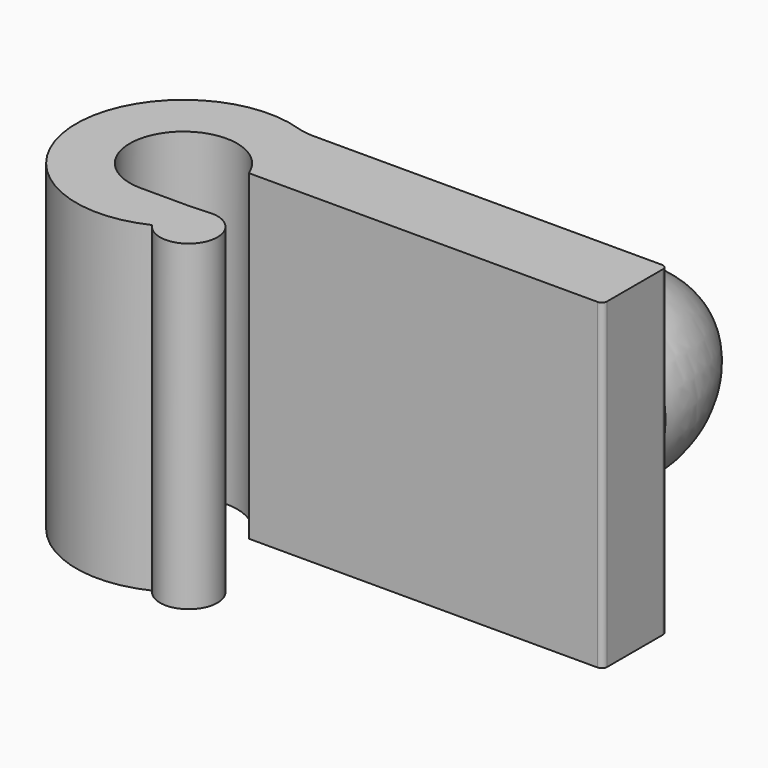
from build123d import *

# Parameters (mm, degrees)
F1_DEPTH      = 6
F3_ANGLE_BACK = 90
F3_ANGLE      = 180


with BuildPart() as f1:
    # F0 (on Top) → F1 (new body, symmetric)
    with BuildSketch(Plane.XY):
        with BuildLine():
            ThreePointArc((0, -2), (-1.6442370944, 1.1386326789), (1.8721820875, 0.7035156225))
            Line((1.8721820875, 0.7035156225), (14.8721820875, 0.7035156225))
            ThreePointArc((14.8721820875, 0.7035156225), (15.0136034438, 0.7620942663), (15.0721820875, 0.9035156225))
            Line((15.0721820875, 0.9035156225), (15.0721820875, 3.5035156225))
            ThreePointArc((15.0721820875, 3.5035156225), (15.0136034438, 3.6449369788), (14.8721820875, 3.7035156225))
            Line((14.8721820875, 3.7035156225), (1.862769321, 3.7035156225))
            ThreePointArc((1.862769321, 3.7035156225), (1.5483999112, 3.7283771782), (1.241846214, 3.8023437484))
            ThreePointArc((1.241846214, 3.8023437484), (-3.9916974669, -0.2575875245), (1.7202481264, -3.6111973615))
            ThreePointArc((1.7202481264, -3.6111973615), (3.5326583833, -3.5785651754), (2.7160516219, -1.9602175008))
            Line((2.7160516219, -1.9602175008), (1.7683124133, -2))
            Line((1.7683124133, -2), (0, -2))
        make_face()
        with BuildLine():
            ThreePointArc((1.7372298538, -3.603058761), (1.7287437795, -3.6071380546), (1.7202481264, -3.6111973615))
            ThreePointArc((1.7202481264, -3.6111973615), (1.7150951564, -3.6032338331), (1.7100129663, -3.5952249487))
            ThreePointArc((1.7100129663, -3.5952249487), (1.7338791511, -3.5635035507), (1.7372298538, -3.603058761))
        make_face(mode=Mode.SUBTRACT)
        with BuildLine():
            ThreePointArc((1.7100129663, -3.5952249487), (1.7150951564, -3.6032338331), (1.7202481264, -3.6111973615))
            ThreePointArc((1.7202481264, -3.6111973615), (1.7287437795, -3.6071380546), (1.7372298538, -3.603058761))
            ThreePointArc((1.7372298538, -3.603058761), (1.7338791511, -3.5635035507), (1.7100129663, -3.5952249487))
        make_face()
    extrude(amount=F1_DEPTH, both=True)



with BuildPart() as f3:
    # F2 (on Top) → F3 (revolve)
    with BuildSketch(Plane.XY, mode=Mode.PRIVATE) as f3_sk:
        with BuildLine():
            Line((7.0616400183, 3.641272106), (9.5616400183, 3.641272106))
            Line((9.5616400183, 3.641272106), (9.5616400183, 10.641272106))
            ThreePointArc((9.5616400183, 10.641272106), (6.8992694056, 8.4986944736), (6.2616400183, 5.141272106))
            Line((6.2616400183, 5.141272106), (7.0616400183, 5.141272106))
            Line((7.0616400183, 5.141272106), (7.0616400183, 3.641272106))
        make_face()
    revolve(f3_sk.sketch.rotate(Axis((9.5616400183, 7.141272106, 0), (0, 1, 0)), -F3_ANGLE_BACK), axis=Axis((9.5616400183, 7.141272106, 0), (0, 1, 0)), revolution_arc=F3_ANGLE)


with BuildPart() as f1_1:
    add(f1.part)

    add(f3.part)  # F5 merges F3
    # F5: F3 across plane
    add(f3.part.mirror(Plane(origin=(10.0616400183, 6.7711546948, 0), x_dir=(0, 1, 0), z_dir=(1, 0, 0))))


solid = f1_1.part
